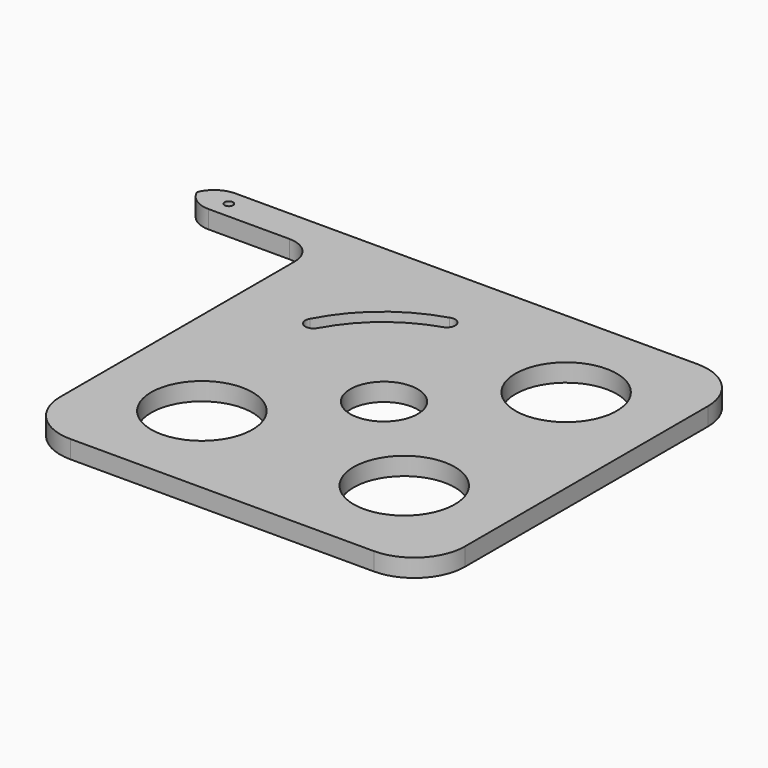
from build123d import *

# Parameters (mm, degrees)
F0_W        = 25.4
F0_H        = 6.35
F1_DEPTH    = 3.3782
F2_D        = 12.7
F3_D        = 19.05
F4_D        = 1.5875
F5_R        = 9.525
F6_T1_DEPTH = 28.7782
F7_R        = 5.08


# Not quite as in the source:
# - a fillet or chamfer that OpenCascade refuses, or shapes differently, is made with other operations: its cross-section is extruded or revolved along the edge and cut away or added
# - a feature names something its author has since deleted; it is built from what else it names


with BuildPart() as f1:
    # F0 (on Top) → F1 (new body)
    with BuildSketch(Plane.XY):
        Polygon((30.6859308559, 40.6974393192), (-45.5140691441, 40.6974393192), (-45.5140691441, 34.3474393192), (-45.5140691441, -35.5025606808), (30.6859308559, -35.5025606808), align=None)
        with BuildLine():
            ThreePointArc((-16.5807714399, 29.4836296191), (-15.0751376879, 29.3583825497), (-14.3562023103, 28.0295666307))
            ThreePointArc((-14.3562023103, 28.0295666307), (-14.7013947794, 27.0412204117), (-15.5868520724, 26.4826942515))
            ThreePointArc((-15.5868520724, 26.4826942515), (-23.6844276087, 22.0164519839), (-29.5755584989, 14.8881544036))
            ThreePointArc((-29.5755584989, 14.8881544036), (-31.7676732764, 14.1678257415), (-32.3633731557, 16.397036865))
            ThreePointArc((-32.3633731557, 16.397036865), (-25.8037717935, 24.5463802201), (-16.5807714399, 29.4836296191))
        make_face(mode=Mode.SUBTRACT)
        with Locations((-58.2140691441, 37.5224393192)):
            Rectangle(F0_W, F0_H)
    extrude(amount=F1_DEPTH)

    # F2 (through all)
    with Locations(Plane(origin=(0, 0, 0), x_dir=(1, 0, 0), z_dir=(0, 0, -1))):
        with Locations((-7.4140691441, -2.5974393192)):
            Hole(F2_D / 2)

    # F3 (through all)
    with Locations(Plane(origin=(0, 0, 0), x_dir=(1, 0, 0), z_dir=(0, 0, -1))):
        with Locations((11.6359308559, -21.6474393192), (11.6359308559, 16.4525606808), (-26.4640691441, 16.4525606808)):
            Hole(F3_D / 2)

    # F4 (through all)
    with Locations(Plane(origin=(0, 0, 0), x_dir=(1, 0, 0), z_dir=(0, 0, -1))):
        with Locations((-64.5640691441, -37.5224393192)):
            Hole(F4_D / 2)

    # F5
    f5_edges = [f1.edges().sort_by_distance(p)[0] for p in [
        (30.685931, -35.502561, 1.6891),
        (-45.514069, -35.502561, 1.6891),
        (30.685931, 40.697439, 1.6891),
    ]]
    fillet(f5_edges, radius=F5_R)

    # F6: fillet of radius 5.08 on 2 edges, made by hand

    # F6_s2 → F6_t1 (cut)
    with BuildSketch(Plane.XY.offset(-12.7)):
        with BuildLine():
            ThreePointArc((-70.9140691441, 35.6174393192), (-69.4261715925, 39.2095417676), (-65.8340691441, 40.6974393192))
            Line((-65.8340691441, 40.6974393192), (-70.9140691441, 40.6974393192))
            Line((-70.9140691441, 40.6974393192), (-70.9140691441, 35.6174393192))
        make_face()
        with BuildLine():
            ThreePointArc((-65.8340691441, 34.3474393192), (-69.4261715925, 35.8353368707), (-70.9140691441, 39.4274393192))
            Line((-70.9140691441, 39.4274393192), (-70.9140691441, 34.3474393192))
            Line((-70.9140691441, 34.3474393192), (-65.8340691441, 34.3474393192))
        make_face()
    extrude(amount=F6_T1_DEPTH, mode=Mode.SUBTRACT)

    # F7
    f7_edges = [f1.edges().sort_by_distance(p)[0] for p in [
        (-45.514069, 34.347439, 1.6891),
    ]]
    fillet(f7_edges, radius=F7_R)


solid = f1.part
